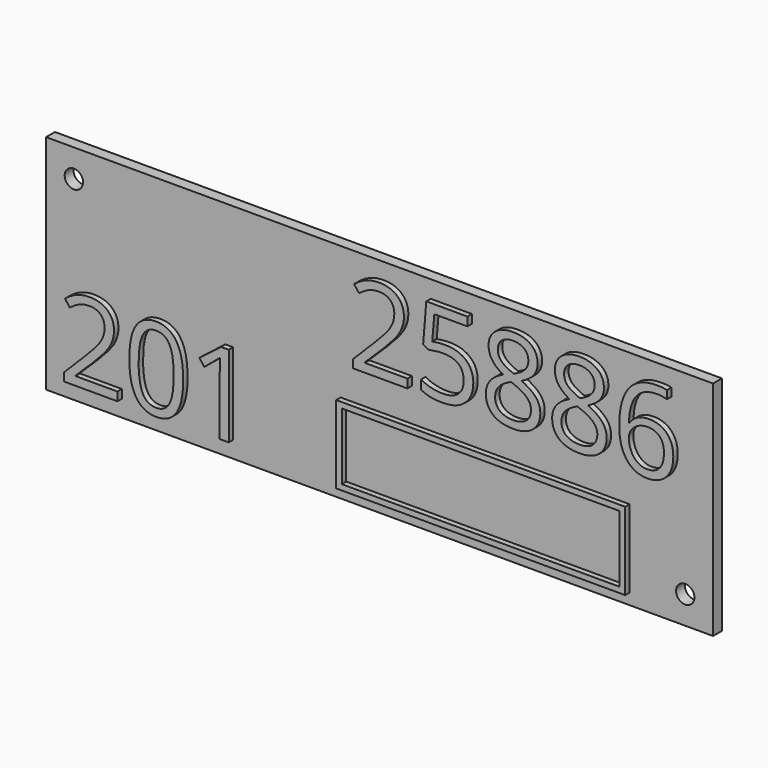
from build123d import *

# Parameters (mm, degrees)
F0_W         = 120
F0_H         = 40
F1_DEPTH     = 2
F3_D         = 3.3
F4_TEXT_SIZE = 20.871833895
F5_DEPTH     = 1
F6_TEXT_SIZE = 20.5478077656
F7_DEPTH     = 1
F8_W         = 52
F8_H         = 14
F8_W_2       = 49.99999962
F8_H_2       = 11.99999962
F9_DEPTH     = 1


# Not quite as in the source:
# - Text() gives the source's letters only with a copy of the font that has no kerning and outlines rounded to 1/6400 em; it was checked with that copy


with BuildPart() as f1:
    # F0 (on Front) → F1 (new body)
    with BuildSketch(Plane.XZ):
        Rectangle(F0_W, F0_H)
    extrude(amount=F1_DEPTH)

    # F3 (through all)
    with Locations(Plane.XZ.offset(2)):
        with Locations((-55, 15), (55, -15)):
            Hole(F3_D / 2)

    # F4 (on face) → F5 (join)
    with BuildSketch(Plane.XZ.offset(2)):
        with Locations((-5, 2)):
            Text('25886', F4_TEXT_SIZE, font='Open Sans', text_align=(TextAlign.LEFT, TextAlign.BOTTOM))
    extrude(amount=F5_DEPTH)

    # F6 (on face) → F7 (join)
    with BuildSketch(Plane.XZ.offset(2)):
        with Locations((-57, -17)):
            Text('201', F6_TEXT_SIZE, font='Open Sans', text_align=(TextAlign.LEFT, TextAlign.BOTTOM))
    extrude(amount=F7_DEPTH)

    # F8 (on face) → F9 (join)
    with BuildSketch(Plane.XZ.offset(2)):
        with Locations((19, -11)):
            Rectangle(F8_W, F8_H)
        with Locations((19, -11)):
            Rectangle(F8_W_2, F8_H_2, mode=Mode.SUBTRACT)
    extrude(amount=F9_DEPTH)


solid = f1.part
